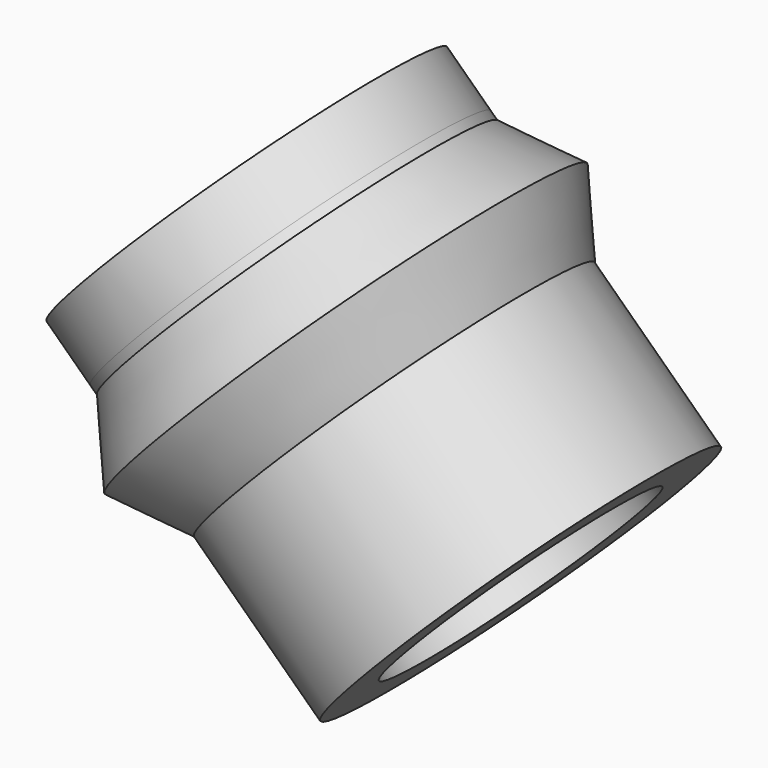
from build123d import *

# Parameters (mm, degrees)
F2_DEPTH = 38
F3_DEPTH = 95
F4_DEPTH = 173


with BuildPart() as f1:
    # F0 (on Front) → F1 (revolve)
    with BuildSketch(Plane.XZ):
        Polygon((-107.8225609797, -15.1899719095), (-86.9944029931, 6.4920546009), (-102.8459925252, 21.7193863706), (-126.1271058847, 14.9773151046), (-154.155441743, 41.9018559024), (-160.4421672051, 35.3574006403), (-148.7241336666, -5.106257544), align=None)
    revolve(axis=Axis((-51.4125548803, 0, 73.4122700717), (0.7211644127, 0, -0.6927639496)))


with BuildPart() as f1b:
    # F0 (on Front) → F1, piece 2 (revolve)
    with BuildSketch(Plane.XZ):
        Polygon((-107.0246264672, 76.2838601884), (-89.8722972673, 81.2510721966), (-105.9747368764, 96.7193752164), (-146.4081794357, 85.0100919422), (-156.4843639398, 44.1390618864), (-154.155441743, 41.9018559024), (-131.2586280567, 65.7373444592), (-110.8642921288, 60.709404342), align=None)
    revolve(axis=Axis((-51.4125548803, 0, 73.4122700717), (0.7211644127, 0, -0.6927639496)))


with BuildPart() as f1c:
    # F0 (on Front) → F1, piece 3 (revolve)
    with BuildSketch(Plane.XZ):
        Polygon((-46.3101103569, 17.9603666249), (-36.2339258527, 58.8313966808), (-66.5911839079, 87.9931434625), (-89.8722972673, 81.2510721966), (-75.6174788212, 67.5576284346), (-83.9806131832, 33.6350741456), (-78.6390218312, 15.1899719095), (-86.9944029931, 6.4920546009), (-86.7435529162, 6.2510833508), align=None)
    revolve(axis=Axis((-51.4125548803, 0, 73.4122700717), (0.7211644127, 0, -0.6927639496)))


with BuildPart() as f2:
    # F2 (new): a face of the model
    f2_faces = [f1.part.faces().sort_by_distance(p)[0] for p in [
        (-22.0355853047, 0, 179.4380812225),
    ]]
    extrude(f2_faces, amount=F2_DEPTH)


with BuildPart() as f3:
    # F3 (new): a face of the model
    f3_faces = [f1.part.faces().sort_by_distance(p)[0] for p in [
        (32.8352718578, 0, 131.2342516077),
    ]]
    extrude(f3_faces, amount=F3_DEPTH)


with BuildPart() as f4:
    # F4 (new): a face of the model
    f4_faces = [f3.part.faces().sort_by_distance(p)[0] for p in [
        (101.345891061, 0, 65.421676393),
    ]]
    extrude(f4_faces, amount=-F4_DEPTH)


solid = Compound([f1.part, f1b.part, f1c.part, f2.part, f3.part, f4.part])
